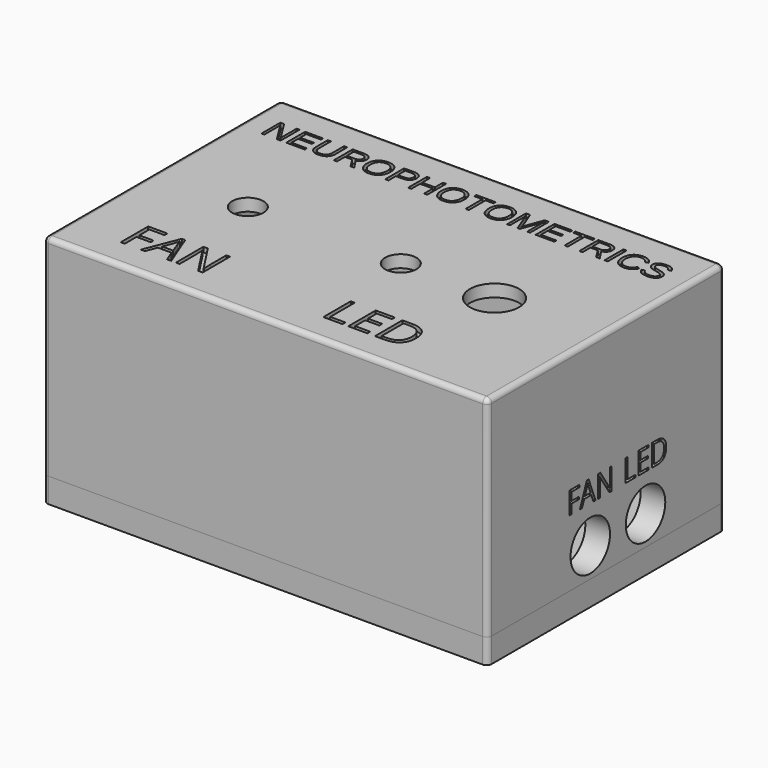
from build123d import *

# Parameters (mm, degrees)
F0_W             = 90
F0_H             = 60
F0_R             = 3.175
F0_R_2           = 5
F1_DEPTH         = 2.5
F2_W             = 90
F2_H             = 60
F2_W_2           = 80
F2_H_2           = 50
F3_DEPTH         = 40
F4_W             = 90
F4_H             = 60
F4_W_2           = 80
F4_H_2           = 50
F5_DEPTH         = 5
F7_D             = 2.4
F7_DEPTH         = 5
F7_CSINK_D       = 4
F7_CSINK_ANGLE   = 90
F7_TIP           = 0.7210327428
F7_2_D           = 2.4
F7_2_DEPTH       = 5
F7_2_CSINK_D     = 4
F7_2_CSINK_ANGLE = 90
F7_2_TIP         = 0.7210327428
F9_D             = 2.9
F9_DEPTH         = 5.2
F9_CBORE_D       = 3.7
F9_CBORE_DEPTH   = 0.2
F9_TIP           = 0.8712478976
F10_R            = 1
F10_2_R          = 1
F11_R            = 5
F12_DEPTH        = 5
F13_R            = 5
F14_DEPTH        = 5
F15_TEXT_SIZE    = 6.9444444444
F16_DEPTH        = 1
F18_TEXT_SIZE    = 9.7222222222
F19_DEPTH        = 1
F20_TEXT_SIZE    = 6.25
F21_DEPTH        = 1
F22_TEXT_SIZE    = 6.25
F23_DEPTH        = 1


# Not quite as in the source:
# - a feature names something its author has since deleted; it is built from what else it names
# - Text() gives the source's letters only with a copy of the font that has no kerning and outlines rounded to 1/6400 em; it was checked with that copy


with BuildPart() as f1:
    # F0 (on Top) → F1 (new body)
    with BuildSketch(Plane.XY):
        with Locations((45, 30)):
            Rectangle(F0_W, F0_H)
        with Locations((19, 28)):
            Circle(F0_R, mode=Mode.SUBTRACT)
        with Locations((50, 28)):
            Circle(F0_R, mode=Mode.SUBTRACT)
        with Locations((69, 28)):
            Circle(F0_R_2, mode=Mode.SUBTRACT)
    extrude(amount=F1_DEPTH)

    # F2 (on face) → F3 (join)
    with BuildSketch(Plane(origin=(0, 0, 0), x_dir=(1, 0, 0), z_dir=(0, 0, -1))):
        with Locations((45, -30)):
            Rectangle(F2_W, F2_H)
        with Locations((45, -30)):
            Rectangle(F2_W_2, F2_H_2, mode=Mode.SUBTRACT)
    extrude(amount=F3_DEPTH)

    # F7
    with Locations(Plane(origin=(0, 0, -45), x_dir=(1, 0, 0), z_dir=(0, 0, -1))):
        with Locations((2.5, -2.5), (2.5, -57.5), (87.5, -57.5), (87.5, -2.5)):
            CounterSinkHole(F7_D / 2, F7_CSINK_D / 2, depth=F7_DEPTH, counter_sink_angle=F7_CSINK_ANGLE)
            with Locations((0, 0, -(F7_DEPTH + F7_TIP / 2))):  # 118° drill point
                Cone(0, F7_D / 2, F7_TIP, mode=Mode.SUBTRACT)

    # F9
    with Locations(Plane(origin=(0, 0, -40), x_dir=(1, 0, 0), z_dir=(0, 0, -1))):
        with Locations((2.5, -2.5), (2.5, -57.5), (87.5, -57.5), (87.5, -2.5)):
            CounterBoreHole(F9_D / 2, F9_CBORE_D / 2, F9_CBORE_DEPTH, depth=F9_DEPTH)
            with Locations((0, 0, -(F9_DEPTH + F9_TIP / 2))):  # 118° drill point
                Cone(0, F9_D / 2, F9_TIP, mode=Mode.SUBTRACT)

    # F10
    f10_edges = [f1.edges().sort_by_distance(p)[0] for p in [
        (45, 0, 2.5),
        (0, 30, 2.5),
        (45, 60, 2.5),
        (90, 30, 2.5),
        (90, 0, -18.75),
        (0, 0, -18.75),
        (90, 60, -18.75),
        (0, 60, -18.75),
    ]]
    fillet(f10_edges, radius=F10_R)

    # F11 (on face) → F12 (cut, through all)
    with BuildSketch(Plane(origin=(0, 0, 0), x_dir=(0, -1, 0), z_dir=(-1, 0, 0))):
        with Locations((-15.5, -34)):
            Circle(F11_R)
    extrude(amount=-F12_DEPTH, mode=Mode.SUBTRACT)

    # F13 (on face) → F14 (cut, through all)
    with BuildSketch(Plane.YZ.offset(90)):
        with Locations((26, -34)):
            Circle(F13_R)
        with Locations((40, -34)):
            Circle(F13_R)
    extrude(amount=-F14_DEPTH, mode=Mode.SUBTRACT)

    # F15 (on face) → F16 (cut)
    with BuildSketch(Plane.XY.offset(2.5)):
        with Locations((4.4080946181, 49)):
            Text('NEUROPHOTOMETRICS', F15_TEXT_SIZE, font='Arimo', text_align=(TextAlign.LEFT, TextAlign.BOTTOM))
    extrude(amount=-F16_DEPTH, mode=Mode.SUBTRACT)

    # F17: union 

    # F18 (on face) → F19 (cut)
    with BuildSketch(Plane.XY.offset(2.5)):
        with Locations((9.9120008681, 6)):
            Text('FAN', F18_TEXT_SIZE, font='Open Sans', text_align=(TextAlign.LEFT, TextAlign.BOTTOM))
        with Locations((50.9612630208, 6)):
            Text('LED', F18_TEXT_SIZE, font='Open Sans', text_align=(TextAlign.LEFT, TextAlign.BOTTOM))
    extrude(amount=-F19_DEPTH, mode=Mode.SUBTRACT)

    # F20 (on face) → F21 (cut)
    with BuildSketch(Plane.YZ.offset(90)):
        with Locations((20.1577148437, -26.5)):
            Text('FAN', F20_TEXT_SIZE, font='Open Sans', text_align=(TextAlign.LEFT, TextAlign.BOTTOM))
        with Locations((34.3500976562, -26.5)):
            Text('LED', F20_TEXT_SIZE, font='Open Sans', text_align=(TextAlign.LEFT, TextAlign.BOTTOM))
    extrude(amount=-F21_DEPTH, mode=Mode.SUBTRACT)

    # F22 (on face) → F23 (cut)
    with BuildSketch(Plane(origin=(0, 0, 0), x_dir=(0, -1, 0), z_dir=(-1, 0, 0))):
        with Locations((-26.5268554687, -26.5)):
            Text('POWER', F22_TEXT_SIZE, font='Open Sans', text_align=(TextAlign.LEFT, TextAlign.BOTTOM))
    extrude(amount=-F23_DEPTH, mode=Mode.SUBTRACT)


with BuildPart() as f5:
    # F4 (on face) → F5 (new body)
    with BuildSketch(Plane(origin=(0, 0, -40), x_dir=(1, 0, 0), z_dir=(0, 0, -1))):
        with Locations((45, -30)):
            Rectangle(F4_W, F4_H)
        with Locations((45, -30)):
            Rectangle(F4_W_2, F4_H_2, mode=Mode.SUBTRACT)
        with Locations((45, -30)):
            Rectangle(F4_W_2, F4_H_2)
    extrude(amount=F5_DEPTH)

    # F7#2
    with Locations(Plane(origin=(0, 0, -45), x_dir=(1, 0, 0), z_dir=(0, 0, -1))):
        with Locations((2.5, -2.5), (2.5, -57.5), (87.5, -57.5), (87.5, -2.5)):
            CounterSinkHole(F7_2_D / 2, F7_2_CSINK_D / 2, depth=F7_2_DEPTH, counter_sink_angle=F7_2_CSINK_ANGLE)
            with Locations((0, 0, -(F7_2_DEPTH + F7_2_TIP / 2))):  # 118° drill point
                Cone(0, F7_2_D / 2, F7_2_TIP, mode=Mode.SUBTRACT)

    # F10#2
    f10_2_edges = [f5.edges().sort_by_distance(p)[0] for p in [
        (0, 60, -42.5),
        (0, 0, -42.5),
        (90, 60, -42.5),
        (90, 0, -42.5),
    ]]
    fillet(f10_2_edges, radius=F10_2_R)


solid = Compound([f1.part, f5.part])
